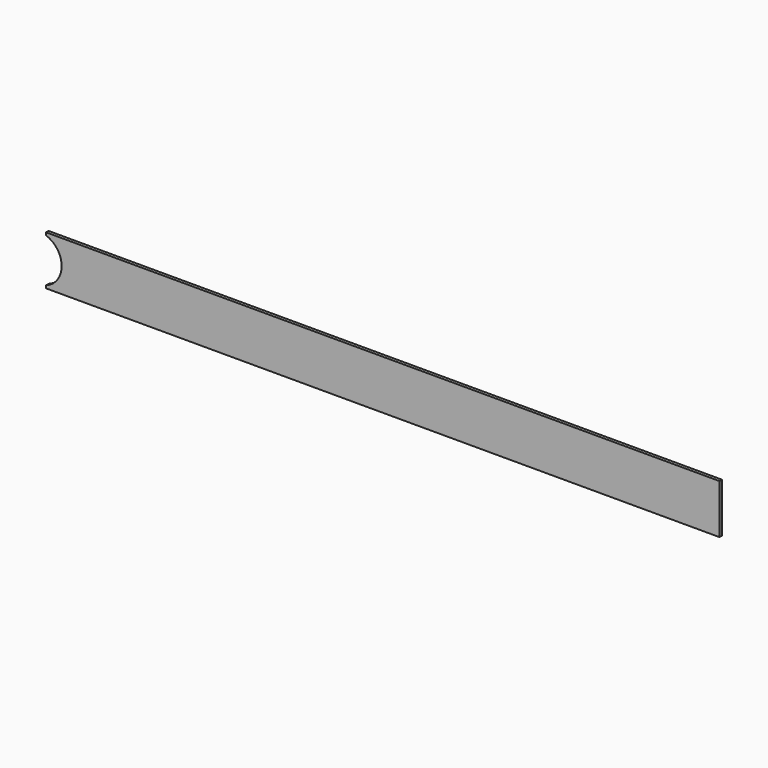
from build123d import *

# Parameters (mm, degrees)
F1_DEPTH = 3.429


# Not quite as in the source:
# - ends of sketch curves that miss each other by under 0.0002 mm in the source are joined


with BuildPart() as f1:
    # F0 (on Front) → F1 (new body)
    with BuildSketch(Plane.XZ):
        with BuildLine():
            Line((882.4181742, 455.9770916), (882.4181742, 509.9520916))
            Line((882.4181742, 509.9520916), (145.8181742, 509.9520916))
            Line((145.8181742, 509.9520916), (145.8181742, 506.941709))
            ThreePointArc((145.8181742, 506.941709), (162.8361742, 482.9645916), (145.818173662, 458.9874757389))
            Line((145.818173662, 458.9874757389), (145.8181742, 455.9770916))
            Line((145.8181742, 455.9770916), (882.4181742, 455.9770916))
        make_face()
    extrude(amount=F1_DEPTH)


solid = f1.part
